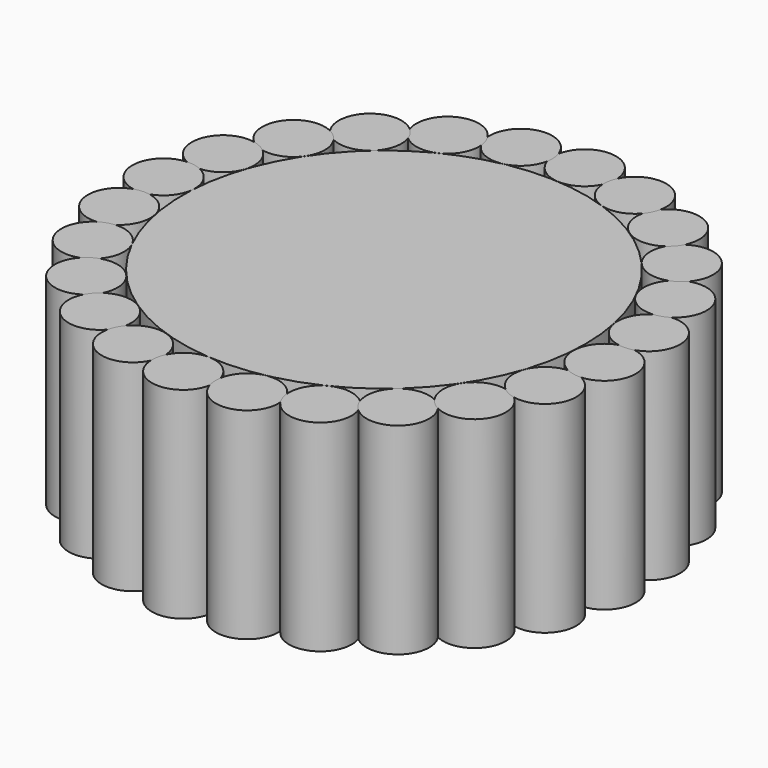
from build123d import *

# Parameters (mm, degrees)
F0_R     = 50
F1_DEPTH = 50
F2_R     = 7.7782886961
F3_DEPTH = 50
F4_COUNT = 24


with BuildPart() as f1:
    # F0 (on Top) → F1 (new body)
    with BuildSketch(Plane.XY):
        Circle(F0_R)
    extrude(amount=F1_DEPTH)


with BuildPart() as f3:
    # F2 (on Top) → F3 (new body)
    with BuildSketch(Plane.XY):
        with Locations((3.697626599, 57.6598491343)):
            Circle(F2_R)
    extrude(amount=F3_DEPTH)


with BuildPart() as f4_1:
    # F4: instance of F3
    add(f3.part.rotate(Axis((0, 0, 50), (0, 0, 1)), 1 * 360 / F4_COUNT))


with BuildPart() as f4_2:
    # F4: instance of F3
    add(f3.part.rotate(Axis((0, 0, 50), (0, 0, 1)), 2 * 360 / F4_COUNT))


with BuildPart() as f4_3:
    # F4: instance of F3
    add(f3.part.rotate(Axis((0, 0, 50), (0, 0, 1)), 3 * 360 / F4_COUNT))


with BuildPart() as f4_4:
    # F4: instance of F3
    add(f3.part.rotate(Axis((0, 0, 50), (0, 0, 1)), 4 * 360 / F4_COUNT))


with BuildPart() as f4_5:
    # F4: instance of F3
    add(f3.part.rotate(Axis((0, 0, 50), (0, 0, 1)), 5 * 360 / F4_COUNT))


with BuildPart() as f4_6:
    # F4: instance of F3
    add(f3.part.rotate(Axis((0, 0, 50), (0, 0, 1)), 6 * 360 / F4_COUNT))


with BuildPart() as f4_7:
    # F4: instance of F3
    add(f3.part.rotate(Axis((0, 0, 50), (0, 0, 1)), 7 * 360 / F4_COUNT))


with BuildPart() as f4_8:
    # F4: instance of F3
    add(f3.part.rotate(Axis((0, 0, 50), (0, 0, 1)), 8 * 360 / F4_COUNT))


with BuildPart() as f4_9:
    # F4: instance of F3
    add(f3.part.rotate(Axis((0, 0, 50), (0, 0, 1)), 9 * 360 / F4_COUNT))


with BuildPart() as f4_10:
    # F4: instance of F3
    add(f3.part.rotate(Axis((0, 0, 50), (0, 0, 1)), 10 * 360 / F4_COUNT))


with BuildPart() as f4_11:
    # F4: instance of F3
    add(f3.part.rotate(Axis((0, 0, 50), (0, 0, 1)), 11 * 360 / F4_COUNT))


with BuildPart() as f4_12:
    # F4: instance of F3
    add(f3.part.rotate(Axis((0, 0, 50), (0, 0, 1)), 12 * 360 / F4_COUNT))


with BuildPart() as f4_13:
    # F4: instance of F3
    add(f3.part.rotate(Axis((0, 0, 50), (0, 0, 1)), 13 * 360 / F4_COUNT))


with BuildPart() as f4_14:
    # F4: instance of F3
    add(f3.part.rotate(Axis((0, 0, 50), (0, 0, 1)), 14 * 360 / F4_COUNT))


with BuildPart() as f4_15:
    # F4: instance of F3
    add(f3.part.rotate(Axis((0, 0, 50), (0, 0, 1)), 15 * 360 / F4_COUNT))


with BuildPart() as f4_16:
    # F4: instance of F3
    add(f3.part.rotate(Axis((0, 0, 50), (0, 0, 1)), 16 * 360 / F4_COUNT))


with BuildPart() as f4_17:
    # F4: instance of F3
    add(f3.part.rotate(Axis((0, 0, 50), (0, 0, 1)), 17 * 360 / F4_COUNT))


with BuildPart() as f4_18:
    # F4: instance of F3
    add(f3.part.rotate(Axis((0, 0, 50), (0, 0, 1)), 18 * 360 / F4_COUNT))


with BuildPart() as f4_19:
    # F4: instance of F3
    add(f3.part.rotate(Axis((0, 0, 50), (0, 0, 1)), 19 * 360 / F4_COUNT))


with BuildPart() as f4_20:
    # F4: instance of F3
    add(f3.part.rotate(Axis((0, 0, 50), (0, 0, 1)), 20 * 360 / F4_COUNT))


with BuildPart() as f4_21:
    # F4: instance of F3
    add(f3.part.rotate(Axis((0, 0, 50), (0, 0, 1)), 21 * 360 / F4_COUNT))


with BuildPart() as f4_22:
    # F4: instance of F3
    add(f3.part.rotate(Axis((0, 0, 50), (0, 0, 1)), 22 * 360 / F4_COUNT))


with BuildPart() as f4_23:
    # F4: instance of F3
    add(f3.part.rotate(Axis((0, 0, 50), (0, 0, 1)), 23 * 360 / F4_COUNT))


solid = Compound([f1.part, f3.part, f4_1.part, f4_2.part, f4_3.part, f4_4.part, f4_5.part, f4_6.part, f4_7.part, f4_8.part, f4_9.part, f4_10.part, f4_11.part, f4_12.part, f4_13.part, f4_14.part, f4_15.part, f4_16.part, f4_17.part, f4_18.part, f4_19.part, f4_20.part, f4_21.part, f4_22.part, f4_23.part])
